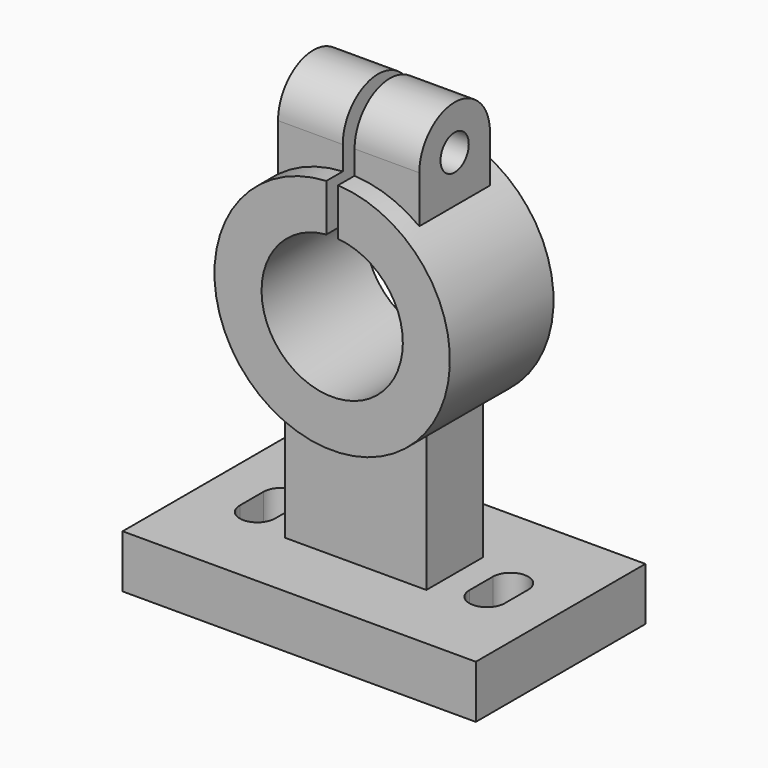
from build123d import *

# Parameters (mm, degrees)
F0_R      = 40
F0_R_2    = 24
F1_DEPTH  = 22
F2_W      = 48
F2_H      = 64
F3_DEPTH  = 12
F4_W      = 120
F4_H      = 72
F5_DEPTH  = 18
F7_DEPTH  = 24
F8_R      = 6
F9_DEPTH  = 84.001
F11_DEPTH = 25
F12_W     = 4
F12_H     = 50
F13_DEPTH = 25


# Not quite as in the source:
# - a pattern or mirror of a feature is missing from the dataset's text; its kind, count and spacing are read off the source's solid


with BuildPart() as f1:
    # F0 (on Front) → F1 (new body, symmetric)
    with BuildSketch(Plane.XZ):
        Circle(F0_R)
        Circle(F0_R_2, mode=Mode.SUBTRACT)
    extrude(amount=F1_DEPTH, both=True)

    # F2 (on Front) → F3 (join, symmetric)
    with BuildSketch(Plane.XZ):
        with Locations((0, -64)):
            Rectangle(F2_W, F2_H)
    extrude(amount=F3_DEPTH, both=True)

    # F4 (on face) → F5 (join)
    with BuildSketch(Plane(origin=(0, 0, -96), x_dir=(1, 0, 0), z_dir=(0, 0, -1))):
        Rectangle(F4_W, F4_H)
    extrude(amount=-F5_DEPTH)

    # F6 (on Right) → F7 (join, symmetric)
    with BuildSketch(Plane.YZ):
        with BuildLine():
            Line((-15, 25), (15, 25))
            Line((15, 25), (15, 48))
            ThreePointArc((15, 48), (0, 63), (-15, 48))
            Line((-15, 48), (-15, 25))
        make_face()
    extrude(amount=F7_DEPTH, both=True)

    # F8 (on face) → F9 (cut, through all)
    with BuildSketch(Plane.YZ.offset(24)):
        with Locations((0, 48)):
            Circle(F8_R)
    extrude(amount=-F9_DEPTH, mode=Mode.SUBTRACT)

    # F10 (on face) → F11 (cut)
    with BuildSketch(Plane(origin=(0, 0, -96), x_dir=(1, 0, 0), z_dir=(0, 0, -1))):
        with BuildLine():
            Line((45, -5), (45, 5))
            ThreePointArc((45, 5), (39, 11), (33, 5))
            Line((33, 5), (33, -5))
            ThreePointArc((33, -5), (39, -11), (45, -5))
        make_face()
    f11 = extrude(amount=-F11_DEPTH, mode=Mode.SUBTRACT)

    # F11_copies: F11 across plane
    add(f11.mirror(Plane(origin=(0, 0, 0), x_dir=(0, 0, -1), z_dir=(-1, 0, 0))), mode=Mode.SUBTRACT)

    # F12 (on Front) → F13 (cut, symmetric)
    with BuildSketch(Plane.XZ):
        with Locations((0, 45)):
            Rectangle(F12_W, F12_H)
    extrude(amount=F13_DEPTH, both=True, mode=Mode.SUBTRACT)


solid = f1.part
